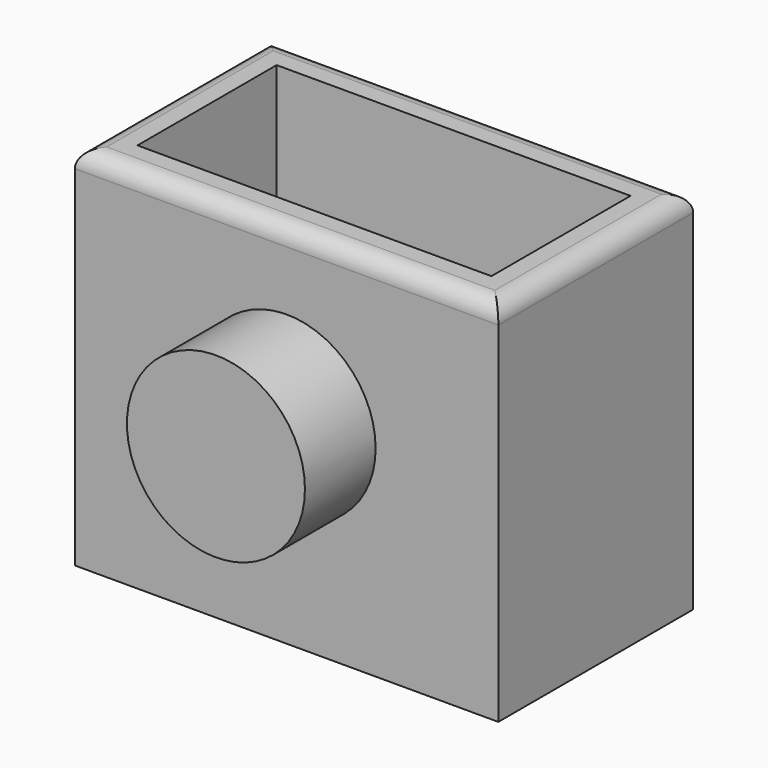
from build123d import *

# Parameters (mm, degrees)
F0_W     = 101.7517447472
F0_H     = 95.5048203468
F1_DEPTH = 25
F2_T     = 10
F3_R     = 25.591656965
F4_DEPTH = 25.4
F5_R     = 5.08


# Not quite as in the source:
# - a pattern or mirror of a feature is missing from the dataset's text; its kind, count and spacing are read off the source's solid


with BuildPart() as f1:
    # F0 (on Front) → F1 (new body, symmetric)
    with BuildSketch(Plane.XZ):
        Rectangle(F0_W, F0_H)
    extrude(amount=F1_DEPTH, both=True)

    # F2
    f2_openings = [f1.faces().sort_by_distance(p)[0] for p in [
        (0, 0, 47.75241),
    ]]
    offset(amount=F2_T, openings=f2_openings, kind=Kind.INTERSECTION)

    # F3 (on face) → F4 (join)
    with BuildSketch(Plane.XZ.offset(35)):
        Circle(F3_R)
    f4 = extrude(amount=F4_DEPTH)

    # F4_copies: F4 across plane
    add(f4.mirror(Plane.ZX))

    # F5
    f5_edges = [f1.edges().sort_by_distance(p)[0] for p in [
        (60.875872, 0, 47.75241),
        (0, 35, 47.75241),
        (-60.875872, 0, 47.75241),
        (0, -35, 47.75241),
    ]]
    fillet(f5_edges, radius=F5_R)


solid = f1.part
